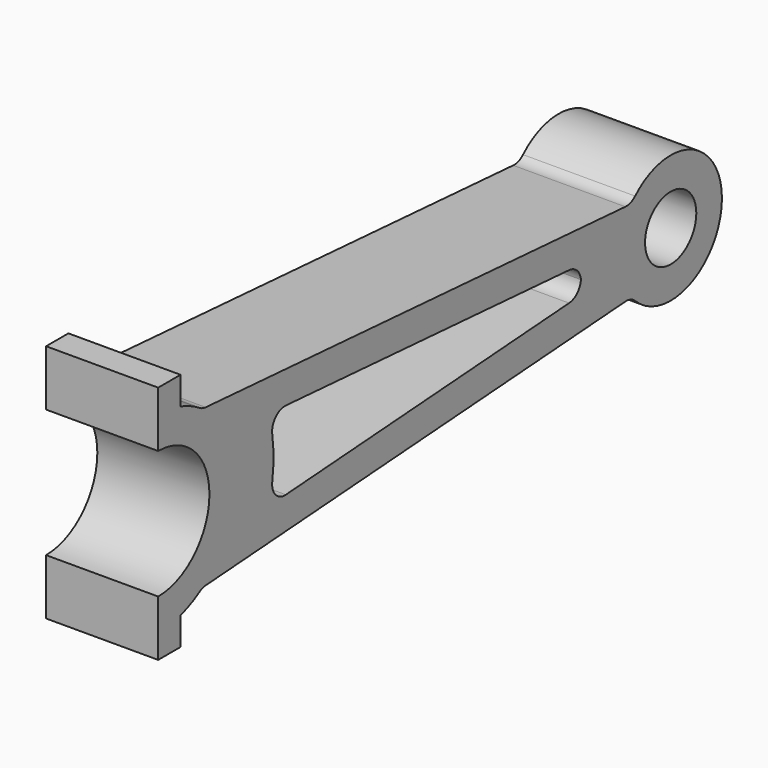
from build123d import *

# Parameters (mm, degrees)
F0_R        = 10
F1_DEPTH    = 35
F2_T1_DEPTH = 35


# Not quite as in the source:
# - a fillet or chamfer that OpenCascade refuses, or shapes differently, is made with other operations: its cross-section is extruded or revolved along the edge and cut away or added


with BuildPart() as f1:
    # F0 (on Right) → F1 (new body)
    with BuildSketch(Plane.YZ):
        with BuildLine():
            Line((17.2200396016, -24.5656311973), (184.6791111376, -12.8557521937))
            ThreePointArc((184.6791111376, -12.8557521937), (220, 0), (184.6791111376, 12.8557521937))
            Line((184.6791111376, 12.8557521937), (17.2200396016, 24.5656311973))
            ThreePointArc((17.2200396016, 24.5656311973), (13.1285920178, 26.9748043854), (8.7082869339, 28.7082869339))
            Line((8.7082869339, 28.7082869339), (8.7082869339, 37.4165738677))
            Line((8.7082869339, 37.4165738677), (0, 37.4165738677))
            Line((0, 37.4165738677), (0, 28.7082869339))
            Line((0, 28.7082869339), (0, 20))
            ThreePointArc((0, 20), (20, 0), (0, -20))
            Line((0, -20), (0, -28.7082869339))
            Line((0, -28.7082869339), (0, -37.4165738677))
            Line((0, -37.4165738677), (8.7082869339, -37.4165738677))
            Line((8.7082869339, -37.4165738677), (8.7082869339, -28.7082869339))
            ThreePointArc((8.7082869339, -28.7082869339), (13.1285920178, -26.9748043854), (17.2200396016, -24.5656311973))
        make_face()
        with BuildLine():
            ThreePointArc((43.1627192329, -12.7271233366), (45, 0), (43.1627192329, 12.7271233366))
            Line((43.1627192329, 12.7271233366), (165.2516861517, 4.1898311065))
            ThreePointArc((165.2516861517, 4.1898311065), (165, 0), (165.2516861517, -4.1898311065))
            Line((165.2516861517, -4.1898311065), (43.1627192329, -12.7271233366))
        make_face(mode=Mode.SUBTRACT)
        with Locations((200, 0)):
            Circle(F0_R, mode=Mode.SUBTRACT)
    extrude(amount=F1_DEPTH)

    # F2: fillet of radius 5 on 8 edges, made by hand

    # F2_s2 → F2_t1 (join)
    with BuildSketch(Plane.YZ):
        with BuildLine():
            ThreePointArc((16.1968645283, 25.2519618931), (17.3232098865, 24.7145443003), (18.547559581, 24.4728019573))
            Line((18.547559581, 24.4728019573), (17.2200396016, 24.5656311973))
            ThreePointArc((17.2200396016, 24.5656311973), (16.7119757319, 24.9140495933), (16.1968645283, 25.2519618931))
        make_face()
        with BuildLine():
            ThreePointArc((182.3113559313, 13.0213217668), (184.3667665167, 13.3094164803), (186.12811064, 14.4073136145))
            ThreePointArc((186.12811064, 14.4073136145), (185.3830095165, 13.6507724765), (184.6791111376, 12.8557521937))
            Line((184.6791111376, 12.8557521937), (182.3113559313, 13.0213217668))
        make_face()
        with BuildLine():
            ThreePointArc((182.3113559313, -13.0213217668), (184.3667665167, -13.3094164803), (186.12811064, -14.4073136145))
            ThreePointArc((186.12811064, -14.4073136145), (185.3830095165, -13.6507724765), (184.6791111376, -12.8557521937))
            Line((184.6791111376, -12.8557521937), (182.3113559313, -13.0213217668))
        make_face()
        with BuildLine():
            ThreePointArc((18.547559581, -24.4728019573), (17.3232098865, -24.7145443003), (16.1968645283, -25.2519618931))
            ThreePointArc((16.1968645283, -25.2519618931), (16.7119757319, -24.9140495933), (17.2200396016, -24.5656311973))
            Line((17.2200396016, -24.5656311973), (18.547559581, -24.4728019573))
        make_face()
        with BuildLine():
            ThreePointArc((160.351373974, 4.5324943146), (163.6398923465, 2.9754237361), (165.0022676546, -0.3984101946))
            ThreePointArc((165.0022676546, -0.3984101946), (165.0515990427, 1.8998080243), (165.2516861517, 4.1898311065))
            Line((165.2516861517, 4.1898311065), (160.351373974, 4.5324943146))
        make_face()
        with BuildLine():
            ThreePointArc((160.351373974, -4.5324943146), (163.6398923465, -2.9754237361), (165.0022676546, 0.3984101946))
            ThreePointArc((165.0022676546, 0.3984101946), (165.0515990427, -1.8998080243), (165.2516861517, -4.1898311065))
            Line((165.2516861517, -4.1898311065), (160.351373974, -4.5324943146))
        make_face()
        with BuildLine():
            ThreePointArc((49.8168417813, 12.2618217605), (45.8004455759, 10.6723259117), (44.5212534713, 6.5466013583))
            ThreePointArc((44.5212534713, 6.5466013583), (43.9507619988, 9.6607722115), (43.1627192329, 12.7271233366))
            Line((43.1627192329, 12.7271233366), (49.8168417813, 12.2618217605))
        make_face()
        with BuildLine():
            ThreePointArc((44.5212534713, -6.5466013583), (45.8004455759, -10.6723259117), (49.8168417813, -12.2618217605))
            Line((49.8168417813, -12.2618217605), (43.1627192329, -12.7271233366))
            ThreePointArc((43.1627192329, -12.7271233366), (43.9507619988, -9.6607722115), (44.5212534713, -6.5466013583))
        make_face()
    extrude(amount=F2_T1_DEPTH)


solid = f1.part
